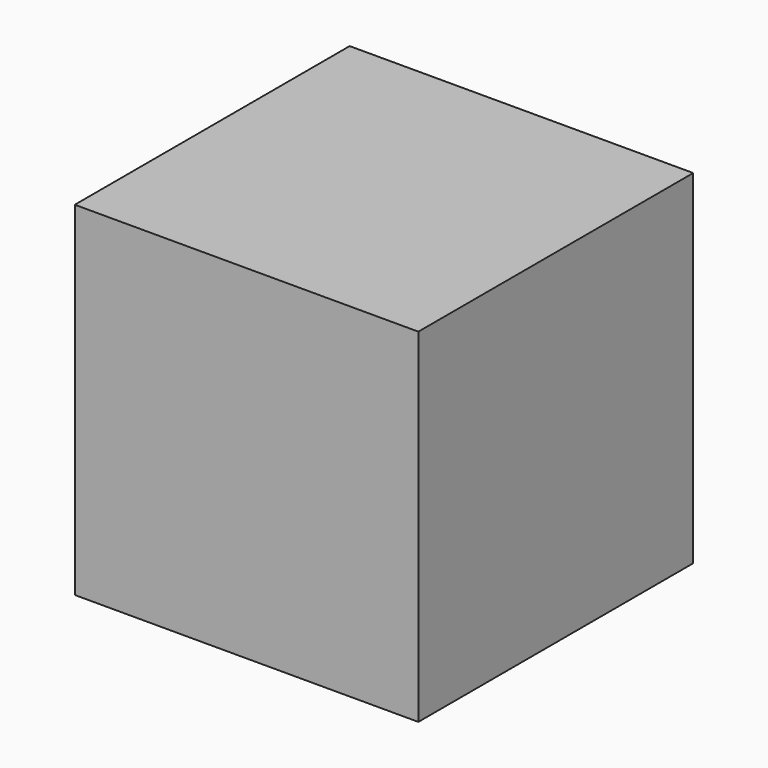
from build123d import *

# Parameters (mm, degrees)
F2_W           = 63.9534269655
F2_H           = 63.9534269655
F3_DEPTH       = 64
F7_W           = 70
F7_H           = 70
F8_DEPTH       = 70
F6_W           = 58.2842652881
F6_H           = 74.5155771047
F9_DEPTH       = 5.7
F9_DEPTH_BACK  = 6
F10_DEPTH      = 6
F10_DEPTH_BACK = 6


with BuildPart() as f3:
    # F2 (on Top) → F3 (new body)
    with BuildSketch(Plane.XY):
        with Locations((-11.9109315234, 3.2196889264)):
            Rectangle(F2_W, F2_H)
    extrude(amount=F3_DEPTH)

    # F7 (on face) → F8 (join)
    with BuildSketch(Plane.XZ.offset(28.7570245564)):
        with Locations((-8.8876450062, 35)):
            Rectangle(F7_W, F7_H)
    extrude(amount=-F8_DEPTH)


with BuildPart() as f9:
    # F6 (on face) → F9 (new body, two sides)
    with BuildSketch(Plane(origin=(-21.9597969133, 0, 21.9438166887), x_dir=(0, 1, 0), z_dir=(0.7073641101, 0, -0.7068493586))) as f9_sk:
        with Locations((6.054269765, 22.1969996005)):
            Rectangle(F6_W, F6_H)
    extrude(amount=F9_DEPTH)
    extrude(f9_sk.sketch, amount=-F9_DEPTH_BACK)

    # F6 (on face) → F10 (join, two sides)
    with BuildSketch(Plane(origin=(-21.9597969133, 0, 21.9438166887), x_dir=(0, 1, 0), z_dir=(0.7073641101, 0, -0.7068493586))) as f10_sk:
        with Locations((6.054269765, 22.1969996005)):
            Rectangle(F6_W, F6_H)
    extrude(amount=F10_DEPTH)
    extrude(f10_sk.sketch, amount=-F10_DEPTH_BACK)


solid = Compound([f3.part, f9.part])
